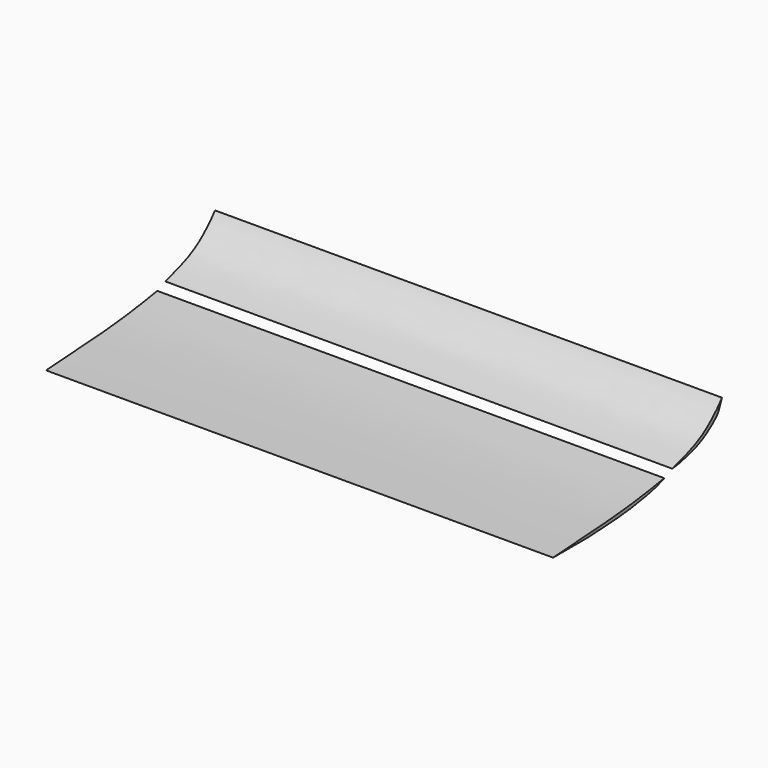
from build123d import *

# Parameters (mm, degrees)
F2_DEPTH = 76.2
F3_DEPTH = 76.2


with BuildPart() as f2:
    # F0 (on Right) → F2 (new body)
    with BuildSketch(Plane.YZ):
        with BuildLine():
            add(Edge.make_bspline(
                [(-20.8933241665, 0), (-16.5957920473, 0.2618400599), (-9.4152230469, 0.6993378063), (-4.0285886841, 1.3634060629), (-1.2735477229, 1.8161906645), (0, 2.0254952833)],
                knots=[0, 0, 0, 0, 0.4449280736, 0.74341195, 1, 1, 1, 1], degree=3))
            Line((-20.8933241665, 0), (-14.3593754619, 0))
            add(Edge.make_bspline(
                [(-14.3593754619, 0), (-13.3347647697, 0.0429284476), (-11.1668279383, 0.1337592025), (-7.1836818354, 0.4373909917), (-4.2718408429, 0.8798975725), (-1.683453406, 1.3580491642), (-0.5254279612, 1.8171765664), (0, 2.0254952833)],
                knots=[0, 0, 0, 0, 0.2115027062, 0.4475109525, 0.6530627628, 0.8425850434, 1, 1, 1, 1], degree=3))
        make_face()
    extrude(amount=F2_DEPTH)


with BuildPart() as f3:
    # F1 (on Right) → F3 (new body)
    with BuildSketch(Plane.YZ):
        with BuildLine():
            add(Edge.make_bspline(
                [(1.5127130318, 2.6591736823), (2.7364566117, 3.03368933), (5.0877174845, 3.7532714412), (7.8124899968, 5.1143543324), (10.1817089845, 7.3960807365), (10.6546288532, 8.0443418411), (10.8260121197, 8.2792676985)],
                knots=[0, 0, 0, 0, 0.2966166535, 0.5699095325, 0.8441378464, 1, 1, 1, 1], degree=3))
            Line((1.5127130318, 2.6591736823), (2.8787299525, 2.8593195602))
            add(Edge.make_bspline(
                [(2.8787299525, 2.8593195602), (3.5485942869, 3.0054688519), (4.9667844391, 3.3148859614), (7.3079096451, 4.1736985069), (9.7433961584, 5.9808127912), (10.1244218897, 6.6280255994), (10.2621791884, 6.8620210513)],
                knots=[0, 0, 0, 0, 0.251047114, 0.5314994792, 0.8306167775, 1, 1, 1, 1], degree=3))
            Line((10.2621791884, 6.8620210513), (10.8260121197, 8.2792676985))
        make_face()
    extrude(amount=F3_DEPTH)


solid = Compound([f2.part, f3.part])
